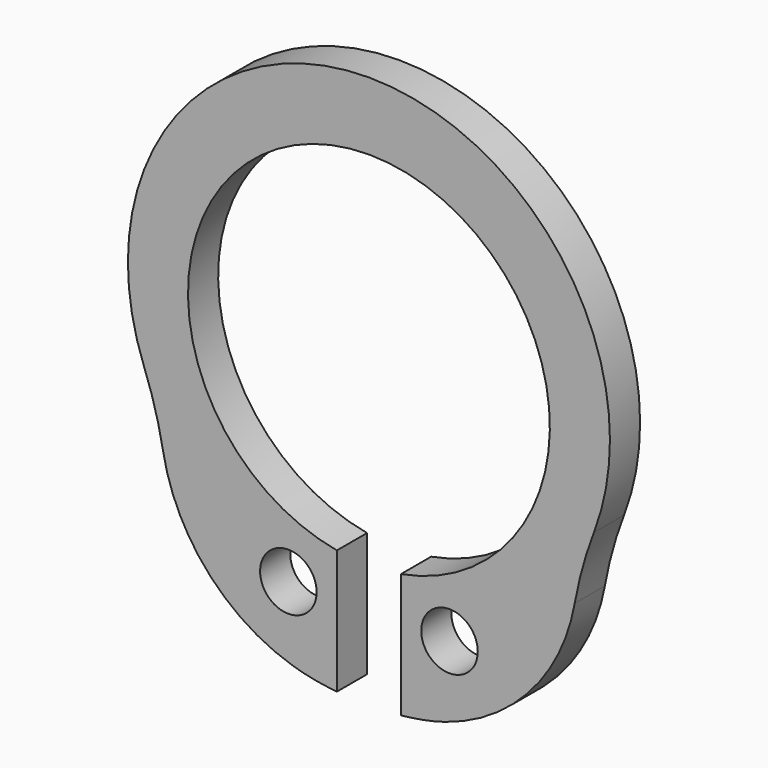
from build123d import *

# Parameters (mm, degrees)
F0_R        = 0.75
F1_DEPTH    = 1
F2_T1_DEPTH = 1
F3_R        = 5


# Not quite as in the source:
# - a fillet or chamfer that OpenCascade refuses, or shapes differently, is made with other operations: its cross-section is extruded or revolved along the edge and cut away or added


with BuildPart() as f1:
    # F0 (on Front) → F1 (new body)
    with BuildSketch(Plane.XZ):
        with BuildLine():
            ThreePointArc((-0.85, -4.7241401334), (0, 4.8), (0.85, -4.7241401334))
            Line((0.85, -4.7241401334), (0.85, -8.0241401334))
            ThreePointArc((0.85, -8.0241401334), (3.2306637909, -7.3940608836), (5.3104097906, -6.0752672975))
            Line((5.3104097906, -6.0752672975), (4.5, -4.3373378932))
            ThreePointArc((4.5, -4.3373378932), (0, 6.6), (-4.5, -4.3373378932))
            Line((-4.5, -4.3373378932), (-5.3104097906, -6.0752672975))
            ThreePointArc((-5.3104097906, -6.0752672975), (-3.2306637909, -7.3940608836), (-0.85, -8.0241401334))
            Line((-0.85, -8.0241401334), (-0.85, -4.7241401334))
        make_face()
        with Locations((-2.1376258958, -5.8730788799)):
            Circle(F0_R, mode=Mode.SUBTRACT)
        with Locations((2.1376258958, -5.8730788799)):
            Circle(F0_R, mode=Mode.SUBTRACT)
    extrude(amount=F1_DEPTH)

    # F2: fillet of radius 10 on 2 edges, made by hand

    # F2_s2 → F2_t1 (join)
    with BuildSketch(Plane.XZ):
        with BuildLine():
            ThreePointArc((-5.9685154732, -2.0889852458), (-5.4360464656, -4.0485437672), (-5.3104097906, -6.0752672975))
            Line((-5.3104097906, -6.0752672975), (-4.5, -4.3373378932))
            ThreePointArc((-4.5, -4.3373378932), (-5.3536180719, -3.2911219818), (-5.9685154732, -2.0889852458))
        make_face()
        with BuildLine():
            ThreePointArc((5.3104097906, -6.0752672975), (5.4360464656, -4.0485437672), (5.9685154732, -2.0889852458))
            ThreePointArc((5.9685154732, -2.0889852458), (5.3536180719, -3.2911219818), (4.5, -4.3373378932))
            Line((4.5, -4.3373378932), (5.3104097906, -6.0752672975))
        make_face()
    extrude(amount=F2_T1_DEPTH)

    # F3
    f3_edges = [f1.edges().sort_by_distance(p)[0] for p in [
        (-5.31041, -0.5, -6.075267),
        (5.31041, -0.5, -6.075267),
    ]]
    fillet(f3_edges, radius=F3_R)


solid = f1.part
